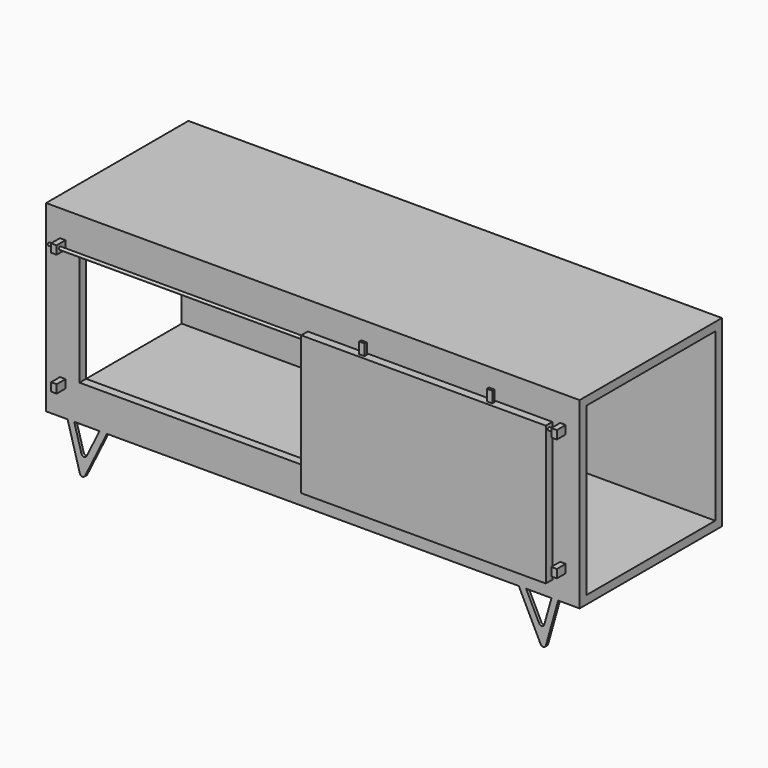
from build123d import *

# Parameters (mm, degrees)
F0_W      = 1219.2
F0_H      = 406.4
F1_DEPTH  = 19.05
F2_W      = 1219.2
F2_H      = 381
F3_DEPTH  = 19.05
F4_W      = 1219.2
F4_H      = 381
F5_DEPTH  = 19.05
F6_W      = 1219.2
F6_H      = 406.4
F7_DEPTH  = 19.05
F8_W      = 12.7
F8_H      = 19.05
F9_DEPTH  = 25.4
F10_R     = 3.175
F11_DEPTH = 1168.4
F13_W     = 558.8
F13_H     = 317.5
F14_DEPTH = 9.398
F15_DEPTH = 9.398
F16_W     = 12.7
F16_H     = 25.4
F17_DEPTH = 3.175
F18_DEPTH = 3.175
F20_DEPTH = 6.35


with BuildPart() as f1:
    # F0 (on Top) → F1 (new body)
    with BuildSketch(Plane.XY):
        Rectangle(F0_W, F0_H)
    extrude(amount=F1_DEPTH)

    # F2 (on face) → F3 (join)
    with BuildSketch(Plane.XZ.offset(203.2)):
        with Locations((0, 209.55)):
            Rectangle(F2_W, F2_H)
        Polygon((-533.4, 336.55), (533.4, 336.55), (533.4, 82.55), (-533.4, 82.55), (-533.4, 209.55), align=None, mode=Mode.SUBTRACT)
    extrude(amount=-F3_DEPTH)

    # F4 (on face) → F5 (join)
    with BuildSketch(Plane(origin=(0, 203.2, 0), x_dir=(-1, 0, 0), z_dir=(0, 1, 0))):
        with Locations((0, 209.55)):
            Rectangle(F4_W, F4_H)
    extrude(amount=-F5_DEPTH)

    # F6 (on face) → F7 (join)
    with BuildSketch(Plane.XY.offset(400.05)):
        Rectangle(F6_W, F6_H)
    extrude(amount=F7_DEPTH)

    # F8 (on face) → F9 (join)
    with BuildSketch(Plane.XZ.offset(203.2)):
        with Locations((-571.5, 349.25)):
            Rectangle(F8_W, F8_H)
        with Locations((571.5, 349.25)):
            Rectangle(F8_W, F8_H)
        with Locations((-571.5, 69.85)):
            Rectangle(F8_W, F8_H)
        with Locations((571.5, 69.85)):
            Rectangle(F8_W, F8_H)
    extrude(amount=F9_DEPTH)

    # F10 (on face) → F11 (join)
    with BuildSketch(Plane.YZ.offset(577.85)):
        with Locations((-219.075, 349.25)):
            Circle(F10_R)
    extrude(amount=-F11_DEPTH)

    # F19 (on face) → F20 (join)
    with BuildSketch(Plane.XZ.offset(203.2)):
        with BuildLine():
            Line((532.4044498456, -99.8943697167), (560.4743361473, 0))
            Line((560.4743361473, 0), (545.3359361473, 0))
            Line((545.3359361473, 0), (528.8258187923, -58.7557694178))
            ThreePointArc((528.8258187923, -58.7557694178), (523.3006211592, -63.3606894596), (517.0209768489, -59.8536729482))
            Line((517.0209768489, -59.8536729482), (487.4107241631, 0))
            Line((487.4107241631, 0), (470.6376492977, 0))
            Line((470.6376492977, 0), (520.5996079022, -100.9922732471))
            ThreePointArc((520.5996079022, -100.9922732471), (526.8792522125, -104.4992897585), (532.4044498456, -99.8943697167))
        make_face()
        with BuildLine():
            Line((-545.3359361473, 0), (-560.4743361473, 0))
            Line((-560.4743361473, 0), (-532.4044498456, -99.8943697167))
            ThreePointArc((-532.4044498456, -99.8943697167), (-526.8792522125, -104.4992897585), (-520.5996079022, -100.9922732471))
            Line((-520.5996079022, -100.9922732471), (-470.6376492977, 0))
            Line((-470.6376492977, 0), (-487.4107241631, 0))
            Line((-487.4107241631, 0), (-517.0209768489, -59.8536729482))
            ThreePointArc((-517.0209768489, -59.8536729482), (-523.3006211592, -63.3606894596), (-528.8258187923, -58.7557694178))
            Line((-528.8258187923, -58.7557694178), (-545.3359361473, 0))
        make_face()
    extrude(amount=-F20_DEPTH)


with BuildPart() as f14:
    # F13 (on offset) → F14 (new body)
    with BuildSketch(Plane.XZ.offset(219.075)):
        with Locations((273.05, 200.66)):
            Rectangle(F13_W, F13_H)
    extrude(amount=F14_DEPTH)

    # F13 (on offset) → F15 (join)
    with BuildSketch(Plane.XZ.offset(219.075)):
        with Locations((273.05, 200.66)):
            Rectangle(F13_W, F13_H)
    extrude(amount=-F15_DEPTH)


with BuildPart() as f17:
    # F16 (on offset) → F17 (new body)
    with BuildSketch(Plane.XZ.offset(219.075)):
        with Locations((127, 372.9595031261)):
            Rectangle(F16_W, F16_H)
    extrude(amount=F17_DEPTH)


with BuildPart() as f17b:
    # F16 (on offset) → F17, piece 2 (new body)
    with BuildSketch(Plane.XZ.offset(219.075)):
        with Locations((419.1, 372.9595031261)):
            Rectangle(F16_W, F16_H)
    extrude(amount=F17_DEPTH)


with BuildPart() as f18:
    # F16 (on offset) → F18 (new body)
    with BuildSketch(Plane.XZ.offset(219.075)):
        with Locations((127, 372.9595031261)):
            Rectangle(F16_W, F16_H)
    extrude(amount=-F18_DEPTH)


with BuildPart() as f18b:
    # F16 (on offset) → F18, piece 2 (new body)
    with BuildSketch(Plane.XZ.offset(219.075)):
        with Locations((419.1, 372.9595031261)):
            Rectangle(F16_W, F16_H)
    extrude(amount=-F18_DEPTH)


solid = Compound([f1.part, f14.part, f17.part, f17b.part, f18.part, f18b.part])
